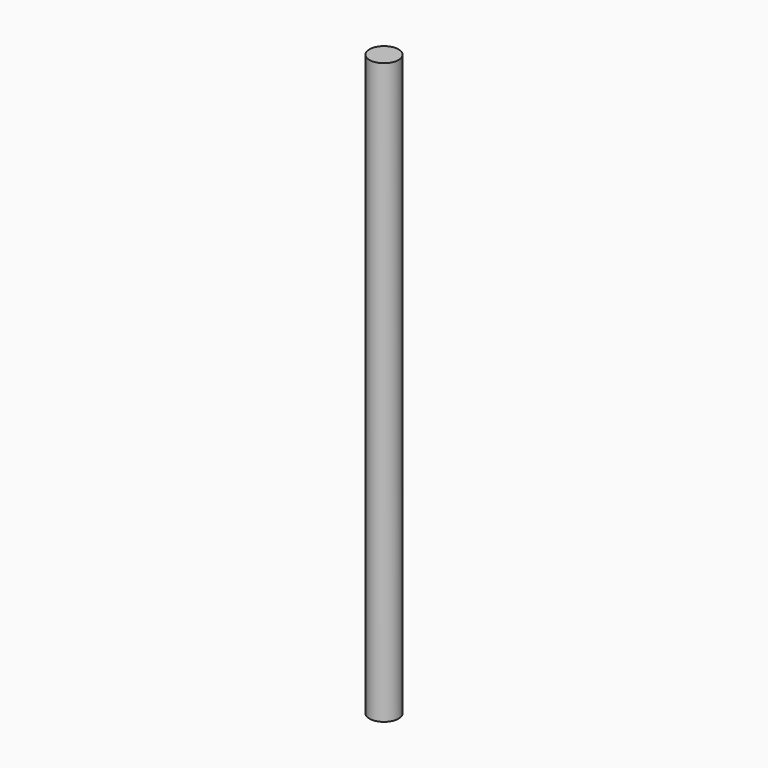
from build123d import *

# Parameters (mm, degrees)
F0_R     = 0.5
F1_DEPTH = 20


# Not quite as in the source:
# - a feature names something its author has since deleted; it is built from what else it names


with BuildPart() as f1:
    # F0 (on Top) → F1 (new body)
    with BuildSketch(Plane.XY):
        Circle(F0_R)
    extrude(amount=F1_DEPTH)


solid = f1.part
